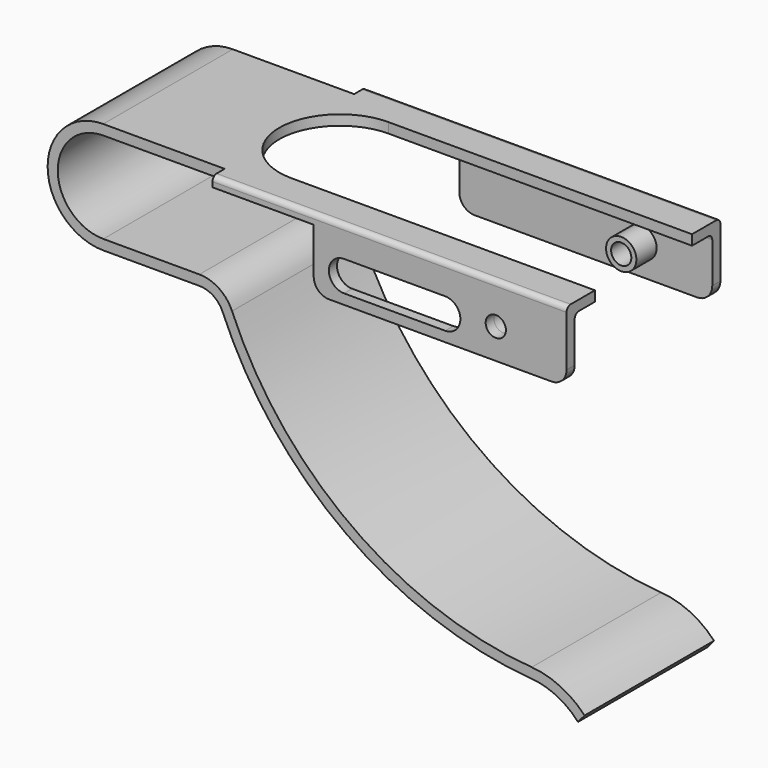
from build123d import *

# Parameters (mm, degrees)
F1_DEPTH  = 16
F2_W      = 70
F2_H      = 3
F3_DEPTH  = 2
F4_W      = 50
F4_H      = 14
F5_DEPTH  = 2
F6_R      = 1
F9_DEPTH  = 2
F11_DEPTH = 25
F13_D     = 4
F13_DEPTH = 50
F13_TIP   = 1.2017212381
F14_R     = 3
F14_R_2   = 2
F15_DEPTH = 5
F16_R     = 3


# Not quite as in the source:
# - a pattern or mirror of a feature is missing from the dataset's text; its kind, count and spacing are read off the source's solid


with BuildPart() as f1:
    # F0 (on Front) → F1 (new body)
    with BuildSketch(Plane.XZ):
        with BuildLine():
            Line((94, 11), (0, 11))
            ThreePointArc((0, 11), (-11, 0), (0, -11))
            Line((0, -11), (19, -11))
            ThreePointArc((19, -11), (21.7681124643, -11.8361612201), (23.6103896104, -14.064978646))
            ThreePointArc((23.6103896104, -14.064978646), (47.8977113224, -44.6078392712), (84.5520957277, -57.9942665386))
            ThreePointArc((84.5520957277, -57.9942665386), (89.6419160729, -59.3768457194), (93.8590048523, -62.5444881493))
            Line((93.8590048523, -62.5444881493), (95.1549842887, -61))
            ThreePointArc((95.1549842887, -61), (90.3976747979, -57.5207528796), (84.7034264019, -56))
            ThreePointArc((84.7034264019, -56), (49.0672193413, -42.9854179344), (25.4545454545, -13.2909701044))
            ThreePointArc((25.4545454545, -13.2909701044), (22.87535745, -10.1706257081), (19, -9))
            Line((19, -9), (0, -9))
            ThreePointArc((0, -9), (-9, 0), (0, 9))
            Line((0, 9), (94, 9))
            Line((94, 9), (94, 11))
        make_face()
    extrude(amount=F1_DEPTH)

    # F2 (on face) → F3 (join)
    with BuildSketch(Plane.XY.offset(11)):
        with Locations((59, -17.5)):
            Rectangle(F2_W, F2_H)
    extrude(amount=-F3_DEPTH)

    # F4 (on face) → F5 (join)
    with BuildSketch(Plane.XZ.offset(19)):
        with Locations((69, 4)):
            Rectangle(F4_W, F4_H)
    extrude(amount=-F5_DEPTH)

    # F6
    f6_edges = [f1.edges().sort_by_distance(p)[0] for p in [
        (59, -19, 11),
        (69, -17, 9),
    ]]
    fillet(f6_edges, radius=F6_R)

    # F7: F1 across plane


with BuildPart() as f1_1:
    add(f1.part)
    add(f1.part.mirror(Plane.XZ))

    # F8 (on face) → F9 (cut)
    with BuildSketch(Plane.XY.offset(11)):
        with BuildLine():
            Line((94, 12), (34, 12))
            ThreePointArc((34, 12), (22, 0), (34, -12))
            Line((34, -12), (94, -12))
            Line((94, -12), (94, 12))
        make_face()
    extrude(amount=-F9_DEPTH, mode=Mode.SUBTRACT)

    # F10 (on face) → F11 (cut)
    with BuildSketch(Plane.XZ.offset(19)):
        with BuildLine():
            ThreePointArc((50, 5), (47, 2), (50, -1))
            Line((50, -1), (70, -1))
            ThreePointArc((70, -1), (73, 2), (70, 5))
            Line((70, 5), (50, 5))
        make_face()
    extrude(amount=-F11_DEPTH, mode=Mode.SUBTRACT)

    # F13
    with Locations(Plane.XZ.offset(19)):
        with Locations((80, 3)):
            Hole(F13_D / 2, depth=F13_DEPTH)
            with Locations((0, 0, -(F13_DEPTH + F13_TIP / 2))):  # 118° drill point
                Cone(0, F13_D / 2, F13_TIP, mode=Mode.SUBTRACT)

    # F14 (on face) → F15 (join)
    with BuildSketch(Plane(origin=(0, -17, 0), x_dir=(-1, 0, 0), z_dir=(0, 1, 0))):
        with Locations((-80, 3)):
            Circle(F14_R)
        with Locations((-80, 3)):
            Circle(F14_R_2, mode=Mode.SUBTRACT)
    f15 = extrude(amount=F15_DEPTH)

    # F15_copies: F15 across plane
    add(f15.mirror(Plane.ZX))

    # F16
    f16_edges = [f1_1.edges().sort_by_distance(p)[0] for p in [
        (94, -18, -3),
        (94, 18, -3),
        (44, -18, -3),
        (44, 18, -3),
    ]]
    fillet(f16_edges, radius=F16_R)


solid = f1_1.part
